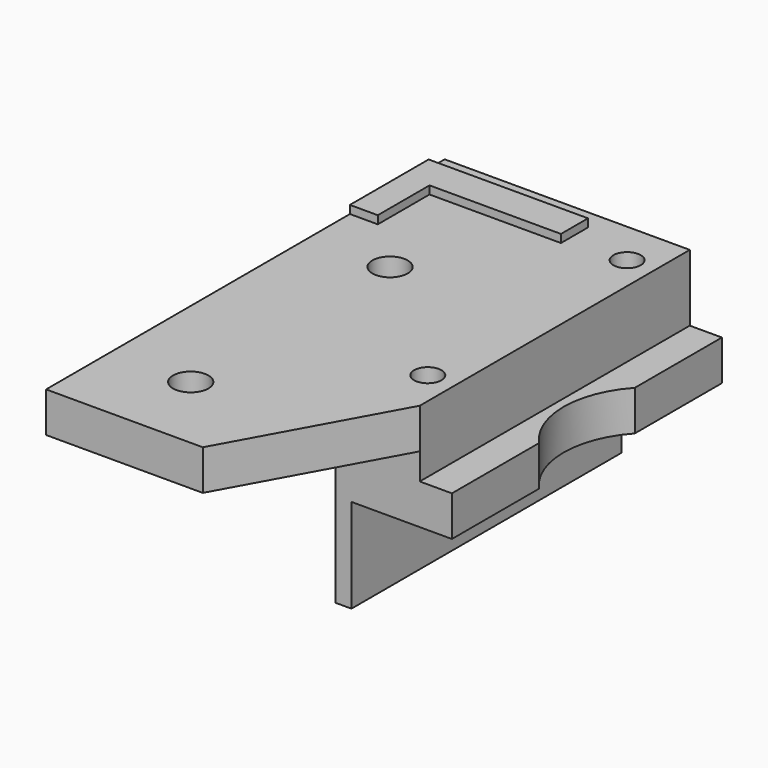
from build123d import *

# Parameters (mm, degrees)
F0_W         = 2
F0_H         = 11.7
F1_DEPTH     = 42
F2_R         = 1.7
F2_R_2       = 11
F3_DEPTH     = 13.301
F4_W         = 62
F4_H         = 5
F5_DEPTH     = 20
F6_R         = 2.2
F7_DEPTH     = 25.001
F8_TEXT_SIZE = 27.7777777778
F9_DEPTH     = 1
F10_DEPTH    = 10.5
F11_SIZE2    = 11
F11_SIZE     = 20


# Not quite as in the source:
# - Text() gives the source's letters only with a copy of the font that has no kerning and outlines rounded to 1/6400 em; it was checked with that copy


with BuildPart() as f1:
    # F0 (on Front) → F1 (new body)
    with BuildSketch(Plane.XZ):
        Polygon((10.5, 5), (10.5, 13.3), (0, 13.3), (0, 0), (2, 0), (14.5, 0), (14.5, 5), align=None)
        with Locations((1, -5.85)):
            Rectangle(F0_W, F0_H)
    extrude(amount=-F1_DEPTH)

    # F2 (on face) → F3 (cut, through all)
    with BuildSketch(Plane(origin=(0, 0, 0), x_dir=(1, 0, 0), z_dir=(0, 0, -1))):
        with Locations((7.1, -5.5)):
            Circle(F2_R)
        with Locations((7.1, -36.5)):
            Circle(F2_R)
        with Locations((22.6, -21)):
            Circle(F2_R_2)
    extrude(amount=-F3_DEPTH, mode=Mode.SUBTRACT)

    # F4 (on face) → F5 (join)
    with BuildSketch(Plane(origin=(0, 0, 0), x_dir=(0, -1, 0), z_dir=(-1, 0, 0))):
        with Locations((-11, 10.8)):
            Rectangle(F4_W, F4_H)
    extrude(amount=F5_DEPTH)

    # F6 (on face) → F7 (cut, through all)
    with BuildSketch(Plane.XY.offset(13.3)):
        with Locations((-10, 21)):
            Circle(F6_R)
        with Locations((-10, -10)):
            Circle(F6_R)
    extrude(amount=-F7_DEPTH, mode=Mode.SUBTRACT)

    # F8 (on face) → F9 (join)
    with BuildSketch(Plane.XY.offset(13.3)):
        with Locations(Location((-20, 42), (0, 0, -90))):
            Text('L', F8_TEXT_SIZE, font='Open Sans', font_style=FontStyle.BOLD, text_align=(TextAlign.LEFT, TextAlign.BOTTOM))
    extrude(amount=F9_DEPTH)

    # F10 (add, through all): a face of the model
    f10_faces = [f1.faces().sort_by_distance(p)[0] for p in [
        (0, -10, 10.8),
    ]]
    extrude(f10_faces, amount=F10_DEPTH)

    # F11
    f11_edges = [f1.edges().sort_by_distance(p)[0] for p in [
        (10.5, -20, 10.8),
    ]]
    f11_side = f1.faces().sort_by_distance((10.5, 14.089612, 9.517811))[0]
    chamfer(f11_edges, length=F11_SIZE, length2=F11_SIZE2, reference=f11_side)


solid = f1.part
